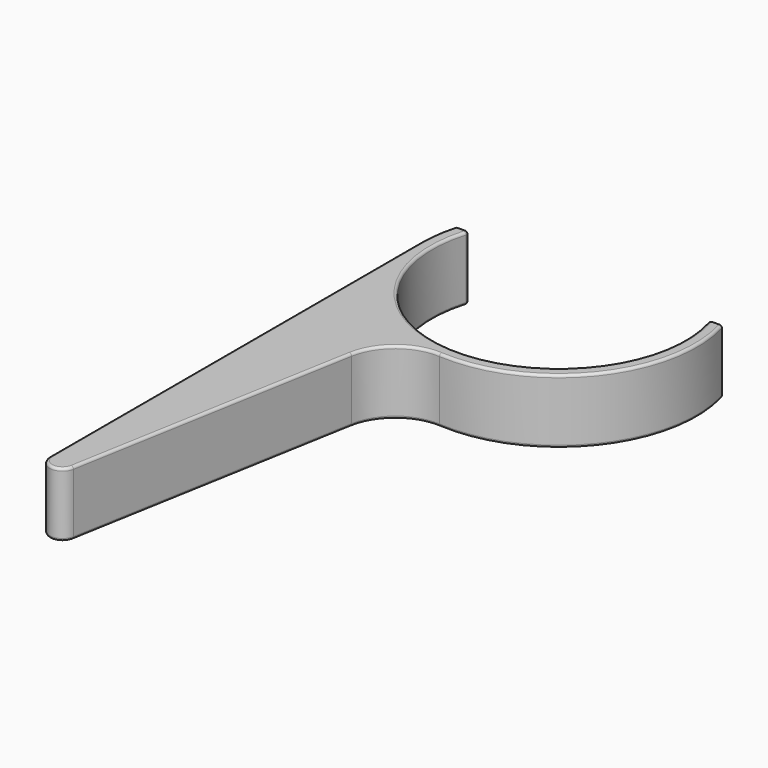
from build123d import *

# Parameters (mm, degrees)
F1_DEPTH = 25
F2_R     = 1


with BuildPart() as f1:
    # F0 (on Top) → F1 (new body)
    with BuildSketch(Plane.XY):
        with BuildLine():
            Line((0, 237.1502615138), (0, 57.1502615138))
            ThreePointArc((0, 57.1502615138), (4.5642212863, 52.1692880233), (9.9240387651, 56.2820206255))
            Line((9.9240387651, 56.2820206255), (29.4444190586, 166.987598496))
            ThreePointArc((29.4444190586, 166.987598496), (36.7733002708, 179.2324763201), (50.3986553344, 183.4750265133))
            ThreePointArc((50.3986553344, 183.4750265133), (95.7512352541, 203.5193518716), (105.4293606826, 252.1502615138))
            Line((105.4293606826, 252.1502615138), (100.4293606826, 252.1502615138))
            ThreePointArc((100.4293606826, 252.1502615138), (53.7817455238, 188.1502615138), (7.134130365, 252.1502615138))
            Line((7.134130365, 252.1502615138), (2.134130365, 252.1502615138))
            ThreePointArc((2.134130365, 252.1502615138), (0.536205584, 244.7257897531), (0, 237.1502615138))
        make_face()
    extrude(amount=F1_DEPTH)

    # F2
    f2_edges = [f1.edges().sort_by_distance(p)[0] for p in [
        (19.684229, 111.63481, 25),
        (102.929361, 252.150262, 25),
        (53.781746, 188.150262, 25),
        (4.63413, 252.150262, 25),
        (0.536206, 244.72579, 25),
        (19.684229, 111.63481, 0),
        (36.7733, 179.232476, 0),
        (95.751235, 203.519352, 0),
        (36.7733, 179.232476, 25),
        (95.751235, 203.519352, 25),
        (102.929361, 252.150262, 0),
        (53.781746, 188.150262, 0),
        (0, 147.150262, 0),
        (4.63413, 252.150262, 0),
        (0.536206, 244.72579, 0),
        (4.564221, 52.169288, 0),
        (105.429361, 252.150262, 12.5),
        (100.429361, 252.150262, 12.5),
        (7.13413, 252.150262, 12.5),
        (2.13413, 252.150262, 12.5),
        (0, 147.150262, 25),
        (4.564221, 52.169288, 25),
    ]]
    fillet(f2_edges, radius=F2_R)


solid = f1.part
